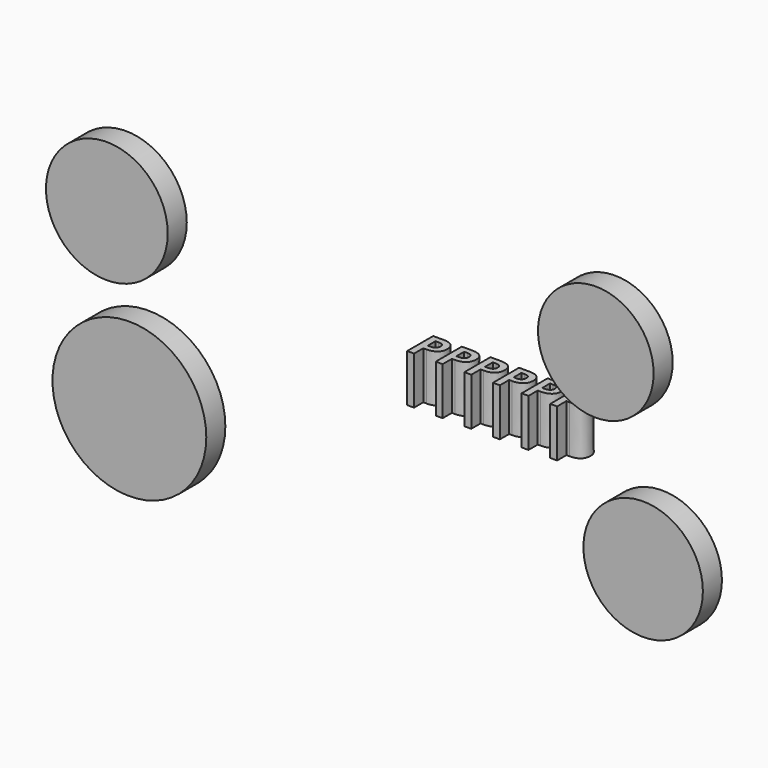
from build123d import *

# Parameters (mm, degrees)
F0_TEXT_SIZE = 24.3016790288
F1_DEPTH     = 25.4
F2_R         = 32.4721526592
F3_DEPTH     = 12.7
F2_R_2       = 41.0216002744
F2_R_3       = 30.8350770826
F2_R_4       = 31.8636621492


# Not quite as in the source:
# - Text() gives the source's letters only with a copy of the font that has no kerning and outlines rounded to 1/6400 em; it was checked with that copy


with BuildPart() as f1:
    # F0 (on Top) → F1 (new body)
    with BuildSketch(Plane.XY):
        with Locations((0, 0)):
            Text('PPPPPP', F0_TEXT_SIZE, font='Open Sans', font_style=FontStyle.BOLD, text_align=(TextAlign.LEFT, TextAlign.BOTTOM))
    extrude(amount=F1_DEPTH)


with BuildPart() as f3:
    # F2 (on Front) → F3 (new body)
    with BuildSketch(Plane.XZ):
        with Locations((-147.8273570538, 47.4730208516)):
            Circle(F2_R)
    extrude(amount=F3_DEPTH)


with BuildPart() as f3b:
    # F2 (on Front) → F3, piece 2 (new body)
    with BuildSketch(Plane.XZ):
        with Locations((-135.8088701963, -41.4637699723)):
            Circle(F2_R_2)
    extrude(amount=F3_DEPTH)


with BuildPart() as f3c:
    # F2 (on Front) → F3, piece 3 (new body)
    with BuildSketch(Plane.XZ):
        with Locations((112.9737496376, 66.1016702652)):
            Circle(F2_R_3)
    extrude(amount=F3_DEPTH)


with BuildPart() as f3d:
    # F2 (on Front) → F3, piece 4 (new body)
    with BuildSketch(Plane.XZ):
        with Locations((138.2125765085, -27.6425089687)):
            Circle(F2_R_4)
    extrude(amount=F3_DEPTH)


solid = Compound([f1.part, f3.part, f3b.part, f3c.part, f3d.part])
